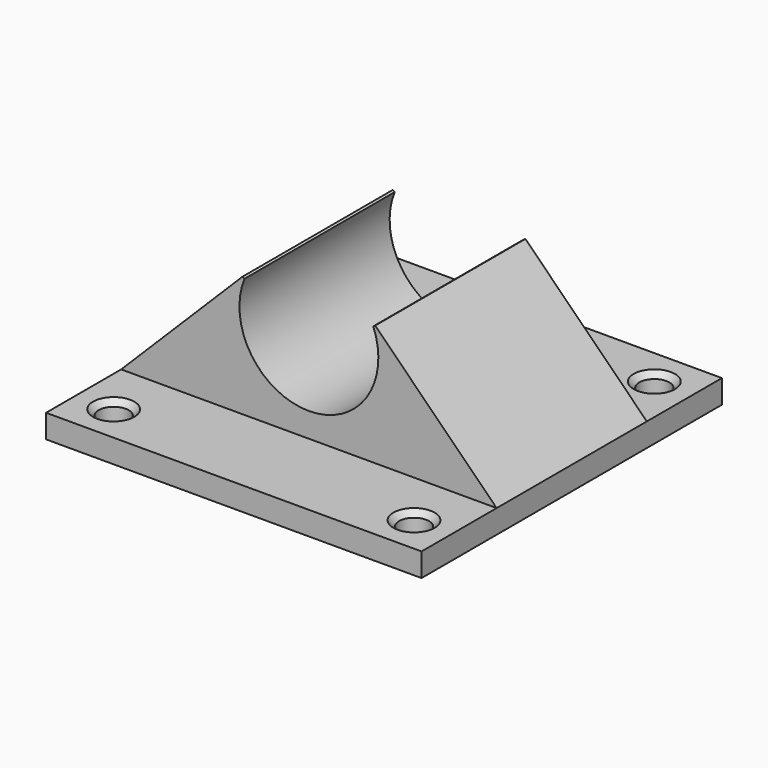
from build123d import *

# Parameters (mm, degrees)
F0_W        = 50.8
F0_H        = 50.8
F1_DEPTH    = 3.175
F3_DEPTH    = 12.7
F4_T1_DEPTH = 29.8470625703
F5_R        = 2.032
F6_DEPTH    = 25.4
F7_SIZE     = 0.762


# Not quite as in the source:
# - a fillet or chamfer that OpenCascade refuses, or shapes differently, is made with other operations: its cross-section is extruded or revolved along the edge and cut away or added


with BuildPart() as f1:
    # F0 (on Top) → F1 (new body)
    with BuildSketch(Plane.XY):
        Rectangle(F0_W, F0_H)
    extrude(amount=F1_DEPTH)

    # F2 (on Front) → F3 (join, symmetric)
    with BuildSketch(Plane.XZ):
        with BuildLine():
            ThreePointArc((8.3472917764, 20.193), (0, 6.477), (-8.3472917764, 20.193))
            Line((-8.3472917764, 20.193), (-25.4, 3.175))
            Line((-25.4, 3.175), (25.4, 3.175))
            Line((25.4, 3.175), (8.3472917764, 20.193))
        make_face()
    extrude(amount=F3_DEPTH, both=True)

    # F4: chamfer of 1.016 on 2 edges, made by hand

    # F4_s2 → F4_t1 (cut)
    with BuildSketch(Plane.XZ.offset(-14.9235312851)):
        with BuildLine():
            Line((-9.00434009, 19.5935484726), (-8.6781133788, 19.3772721718))
            Line((-8.6781133788, 19.3772721718), (-8.659276653, 19.3696511377))
            ThreePointArc((-8.659276653, 19.3696511377), (-8.5217005097, 19.7892691023), (-8.3292435779, 20.1836637838))
            Line((-8.3292435779, 20.1836637838), (-8.3616455415, 20.2073830396))
            ThreePointArc((-8.3616455415, 20.2073830396), (-8.6761048617, 19.893563754), (-9.0186938551, 19.6079315122))
            Line((-9.0186938551, 19.6079315122), (-9.00434009, 19.5935484726))
        make_face()
        with BuildLine():
            Line((9.00434009, 19.5935484726), (8.6781133788, 19.3772721718))
            Line((8.6781133788, 19.3772721718), (8.659276653, 19.3696511377))
            ThreePointArc((8.659276653, 19.3696511377), (8.5217005097, 19.7892691023), (8.3292435779, 20.1836637838))
            Line((8.3292435779, 20.1836637838), (8.3616455415, 20.2073830396))
            ThreePointArc((8.3616455415, 20.2073830396), (8.6761048617, 19.893563754), (9.0186938551, 19.6079315122))
            Line((9.0186938551, 19.6079315122), (9.00434009, 19.5935484726))
        make_face()
    extrude(amount=F4_T1_DEPTH, mode=Mode.SUBTRACT)

    # F5 (on face) → F6 (cut)
    with BuildSketch(Plane(origin=(0, 0, 0), x_dir=(1, 0, 0), z_dir=(0, 0, -1))):
        with Locations((-20.32, 20.32)):
            Circle(F5_R)
        with Locations((-20.32, -20.32)):
            Circle(F5_R)
        with Locations((20.32, 20.32)):
            Circle(F5_R)
        with Locations((20.32, -20.32)):
            Circle(F5_R)
    extrude(amount=-F6_DEPTH, mode=Mode.SUBTRACT)

    # F7
    f7_edges = [f1.edges().sort_by_distance(p)[0] for p in [
        (-22.352, -20.32, 3.175),
        (-22.352, 20.32, 3.175),
        (18.288, 20.32, 3.175),
        (18.288, -20.32, 3.175),
    ]]
    chamfer(f7_edges, length=F7_SIZE)


solid = f1.part
